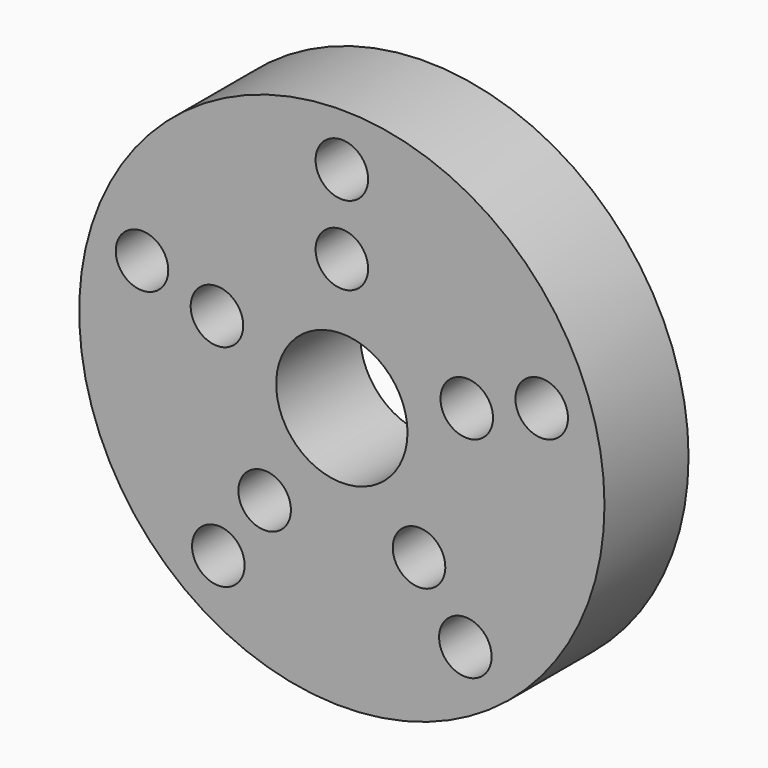
from build123d import *

# Parameters (mm, degrees)
F0_R            = 63.5
F0_R_2          = 15.875
F1_DEPTH        = 25.4
F2_R            = 6.35
F3_DEPTH        = 25.4
F3_COPIES_COUNT = 5


# Not quite as in the source:
# - a pattern or mirror of a feature is missing from the dataset's text; its kind, count and spacing are read off the source's solid


with BuildPart() as f1:
    # F0 (on Front) → F1 (new body)
    with BuildSketch(Plane.XZ):
        Circle(F0_R)
        Circle(F0_R_2, mode=Mode.SUBTRACT)
    extrude(amount=F1_DEPTH)

    # F2 (on face) → F3 (cut, through all)
    with BuildSketch(Plane.XZ.offset(25.4)):
        with Locations((0, 50.8)):
            Circle(F2_R)
        with Locations((0, 31.75)):
            Circle(F2_R)
    f3 = extrude(amount=-F3_DEPTH, mode=Mode.SUBTRACT)

    # F3_copies: F3 ×5 about axis
    f3_copies_axis = Axis((0, 0, 0), (0, 1, 0))
    for i in range(1, F3_COPIES_COUNT):
        add(f3.rotate(f3_copies_axis, i * 360 / F3_COPIES_COUNT), mode=Mode.SUBTRACT)


solid = f1.part
